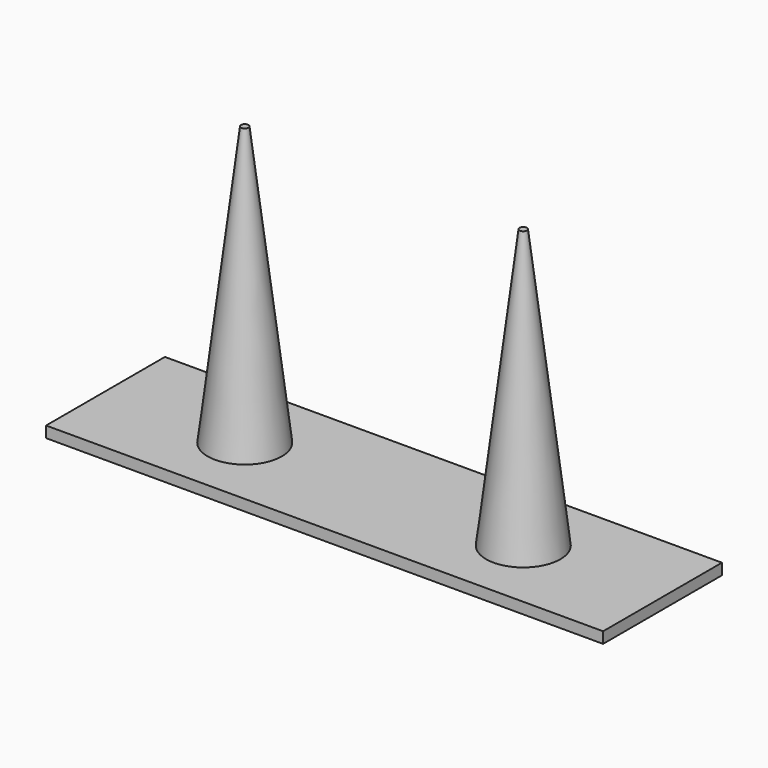
from build123d import *

# Parameters (mm, degrees)
F0_W     = 30
F0_H     = 8
F1_DEPTH = 0.6


# Not quite as in the source:
# - a pattern or mirror of a feature is missing from the dataset's text; its kind, count and spacing are read off the source's solid


with BuildPart() as f1:
    # F0 (on Top) → F1 (new body)
    with BuildSketch(Plane.XY):
        Rectangle(F0_W, F0_H)
    extrude(amount=F1_DEPTH)

    # F2 (on Front) → F3 (revolve)
    with BuildSketch(Plane.XZ):
        Polygon((-5.5, 0.6), (-7.3, 15.6), (-7.5, 15.6), (-7.5, 0.6), align=None)
    f3 = revolve(axis=Axis((-7.5, 0, 8.1), (0, 0, -1)))

    # F3_copies: F3 across plane
    add(f3.mirror(Plane(origin=(0, 0, 0), x_dir=(0, 0, 1), z_dir=(1, 0, 0))))


solid = f1.part
